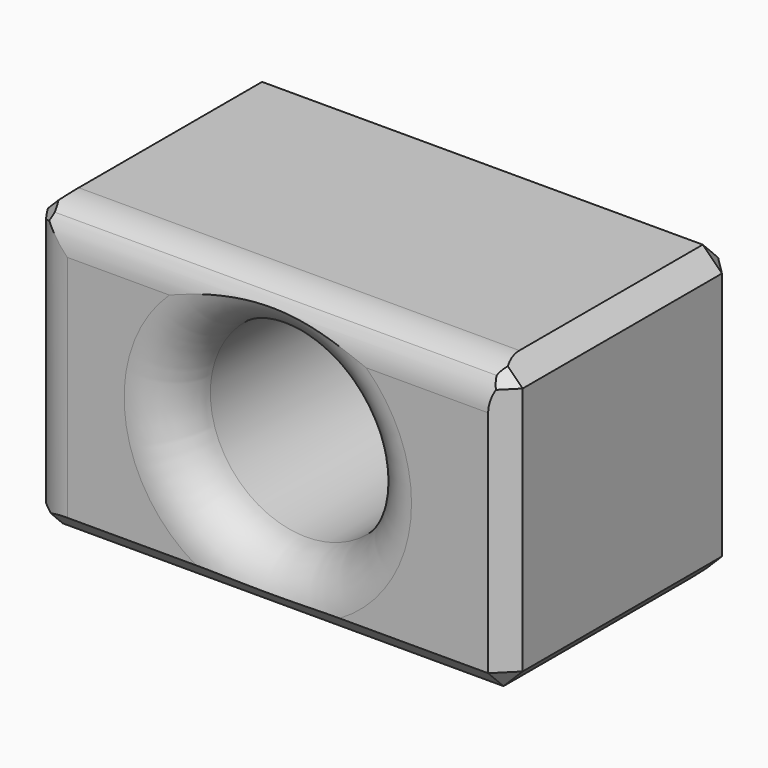
from build123d import *

# Parameters (mm, degrees)
F0_W        = 127
F0_H        = 76.2
F0_R        = 25.4
F1_DEPTH    = 76.2
F2_SIZE     = 5.08
F3_T1_DEPTH = 143.1425612107
F3_T3_DEPTH = 92.3425612107


# Not quite as in the source:
# - a fillet or chamfer that OpenCascade refuses, or shapes differently, is made with other operations: its cross-section is extruded or revolved along the edge and cut away or added


with BuildPart() as f1:
    # F0 (on Front) → F1 (new body)
    with BuildSketch(Plane.XZ):
        Rectangle(F0_W, F0_H)
        Circle(F0_R, mode=Mode.SUBTRACT)
    extrude(amount=F1_DEPTH)

    # F2
    f2_edges = [f1.edges().sort_by_distance(p)[0] for p in [
        (0, -76.2, 38.1),
        (-63.5, -38.1, 38.1),
        (0, 0, 38.1),
        (63.5, -38.1, 38.1),
        (63.5, -76.2, 0),
        (0, -76.2, -38.1),
        (-63.5, -76.2, 0),
        (63.5, -38.1, -38.1),
        (63.5, 0, 0),
        (0, 0, -38.1),
        (-63.5, 0, 0),
        (-63.5, -38.1, -38.1),
    ]]
    chamfer(f2_edges, length=F2_SIZE)

    # F3: fillet of radius 12.7 on 10 edges, made by hand

    # F3_s2 → F3_t1 (cut)
    with BuildSketch(Plane.YZ.offset(-71.5712806053)):
        with BuildLine():
            ThreePointArc((0, -27.7594877579), (-0.9667299371, -32.6195673489), (-3.7197438789, -36.7397438789))
            Line((-3.7197438789, -36.7397438789), (0, -33.02))
            Line((0, -33.02), (0, -27.7594877579))
        make_face()
        with BuildLine():
            ThreePointArc((-1.3602561211, -34.3802561211), (-5.4804326511, -37.1332700629), (-10.3405122421, -38.1))
            Line((-10.3405122421, -38.1), (-5.08, -38.1))
            Line((-5.08, -38.1), (-1.3602561211, -34.3802561211))
        make_face()
        with BuildLine():
            ThreePointArc((-65.8594877579, 38.1), (-70.7195673489, 37.1332700629), (-74.8397438789, 34.3802561211))
            Line((-74.8397438789, 34.3802561211), (-71.12, 38.1))
            Line((-71.12, 38.1), (-65.8594877579, 38.1))
        make_face()
        with BuildLine():
            ThreePointArc((-72.4802561211, 36.7397438789), (-75.2332700629, 32.6195673489), (-76.2, 27.7594877579))
            Line((-76.2, 27.7594877579), (-76.2, 33.02))
            Line((-76.2, 33.02), (-72.4802561211, 36.7397438789))
        make_face()
    extrude(amount=F3_T1_DEPTH, mode=Mode.SUBTRACT)

    # F3_s4 → F3_t3 (cut)
    with BuildSketch(Plane.XY.offset(-46.1712806053)):
        with BuildLine():
            ThreePointArc((-63.5, -65.8594877579), (-62.5332700629, -70.7195673489), (-59.7802561211, -74.8397438789))
            Line((-59.7802561211, -74.8397438789), (-63.5, -71.12))
            Line((-63.5, -71.12), (-63.5, -65.8594877579))
        make_face()
        with BuildLine():
            ThreePointArc((-53.1594877579, -76.2), (-58.0195673489, -75.2332700629), (-62.1397438789, -72.4802561211))
            Line((-62.1397438789, -72.4802561211), (-58.42, -76.2))
            Line((-58.42, -76.2), (-53.1594877579, -76.2))
        make_face()
        with BuildLine():
            ThreePointArc((-63.5, -10.3405122421), (-62.5332700629, -5.4804326511), (-59.7802561211, -1.3602561211))
            Line((-59.7802561211, -1.3602561211), (-63.5, -5.08))
            Line((-63.5, -5.08), (-63.5, -10.3405122421))
        make_face()
        with BuildLine():
            ThreePointArc((-53.1594877579, 0), (-58.0195673489, -0.9667299371), (-62.1397438789, -3.7197438789))
            Line((-62.1397438789, -3.7197438789), (-58.42, 0))
            Line((-58.42, 0), (-53.1594877579, 0))
        make_face()
    extrude(amount=F3_T3_DEPTH, mode=Mode.SUBTRACT)

    # F3_s5 → F3_t6 (revolve, cut)
    with BuildSketch(Plane.XY):
        with BuildLine():
            ThreePointArc((38.1, -76.2), (29.1197438789, -72.4802561211), (25.4, -63.5))
            Line((25.4, -63.5), (25.4, -76.2))
            Line((25.4, -76.2), (38.1, -76.2))
        make_face()
    revolve(axis=Axis((0, -76.2, 0), (0, -1, 0)), mode=Mode.SUBTRACT)

    # F3_s7 → F3_t8 (revolve, cut)
    with BuildSketch(Plane.XY):
        with BuildLine():
            ThreePointArc((38.1, 0), (29.1197438789, -3.7197438789), (25.4, -12.7))
            Line((25.4, -12.7), (25.4, 0))
            Line((25.4, 0), (38.1, 0))
        make_face()
    revolve(axis=Axis((0, 0, 0), (0, -1, 0)), mode=Mode.SUBTRACT)


solid = f1.part
